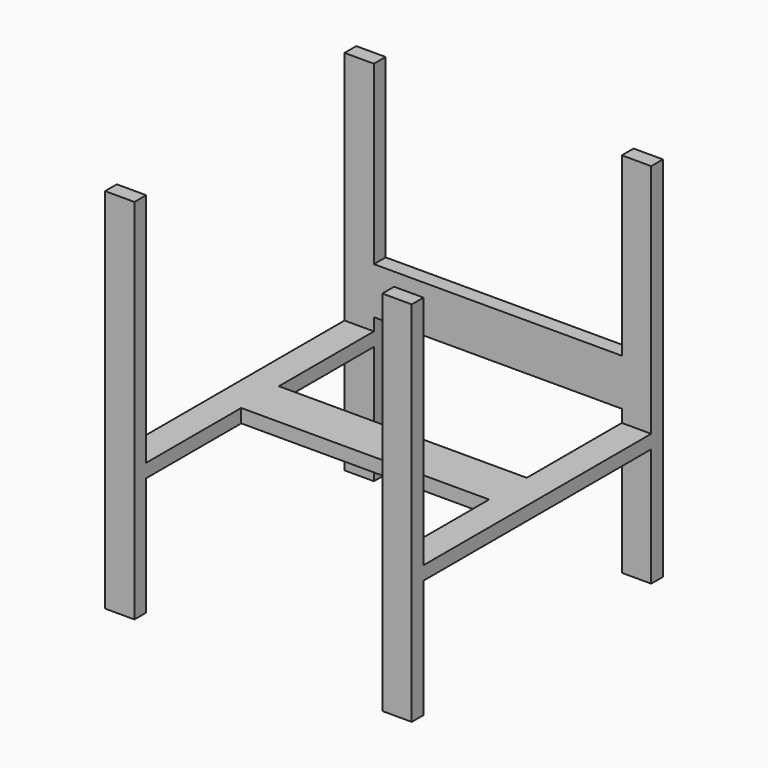
from build123d import *

# Parameters (mm, degrees)
F0_W     = 914.4
F0_H     = 914.4
F0_W_2   = 80
F0_H_2   = 40
F1_DEPTH = 40
F2_DEPTH = 1000
F4_W     = 674.4
F4_H     = 40
F5_DEPTH = 127
F7_W     = 674.4
F7_H     = 128
F8_DEPTH = 37
F9_DEPTH = 40


# Not quite as in the source:
# - a feature names something its author has since deleted; it is built from what else it names


with BuildPart() as f1:
    # F0 (on Top) → F1 (new body)
    with BuildSketch(Plane.XY):
        Rectangle(F0_W, F0_H)
        with Locations((-377.2, -407.2)):
            Rectangle(F0_W_2, F0_H_2, mode=Mode.SUBTRACT)
        with Locations((377.2, -407.2)):
            Rectangle(F0_W_2, F0_H_2, mode=Mode.SUBTRACT)
        with Locations((-377.2, 407.2)):
            Rectangle(F0_W_2, F0_H_2, mode=Mode.SUBTRACT)
        with Locations((377.2, 407.2)):
            Rectangle(F0_W_2, F0_H_2, mode=Mode.SUBTRACT)
        with Locations((-377.2, -407.2)):
            Rectangle(F0_W_2, F0_H_2)
        with Locations((377.2, 407.2)):
            Rectangle(F0_W_2, F0_H_2)
        with Locations((377.2, -407.2)):
            Rectangle(F0_W_2, F0_H_2)
        with Locations((-377.2, 407.2)):
            Rectangle(F0_W_2, F0_H_2)
    extrude(amount=F1_DEPTH)

    # F0 (on Top) → F2 (join)
    with BuildSketch(Plane.XY):
        with Locations((-377.2, -407.2)):
            Rectangle(F0_W_2, F0_H_2)
        with Locations((-377.2, 407.2)):
            Rectangle(F0_W_2, F0_H_2)
        with Locations((377.2, -407.2)):
            Rectangle(F0_W_2, F0_H_2)
        with Locations((377.2, 407.2)):
            Rectangle(F0_W_2, F0_H_2)
    extrude(amount=-F2_DEPTH)

    # F4 (on offset) → F5 (join)
    with BuildSketch(Plane.XY.offset(-607)):
        with Locations((0, 407.2)):
            Rectangle(F4_W, F4_H)
    extrude(amount=F5_DEPTH)

    # F7 (on offset) → F8 (join)
    with BuildSketch(Plane.XY.offset(-678)):
        Polygon((-417.2, 387.2), (-417.2, -387.2), (-337.2, -387.2), (-337.2, -64), (-337.2, 64), (-337.2, 387.2), align=None)
        Polygon((337.2, 64), (337.2, -64), (337.2, -387.2), (417.2, -387.2), (417.2, 387.2), (337.2, 387.2), align=None)
        Rectangle(F7_W, F7_H)
    extrude(amount=F8_DEPTH)

    # F9 (cut): a face of the model
    f9_faces = [f1.faces().sort_by_distance(p)[0] for p in [
        (0, 0, 40),
    ]]
    extrude(f9_faces, amount=-F9_DEPTH, mode=Mode.SUBTRACT)


solid = f1.part
